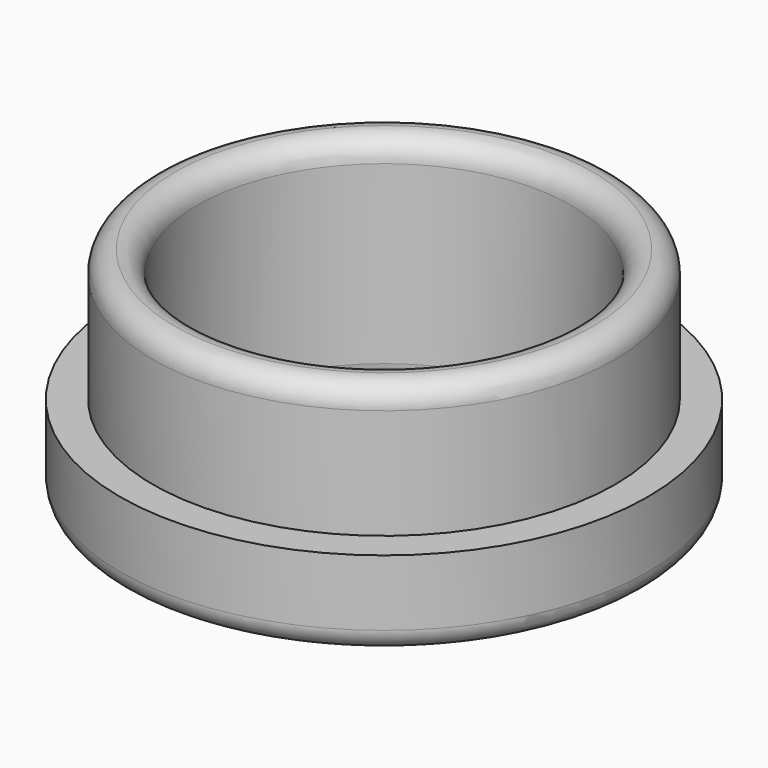
from build123d import *

# Parameters (mm, degrees)
F0_R     = 10.5
F0_R_2   = 8.5
F1_DEPTH = 10
F0_R_3   = 12
F2_DEPTH = 4
F3_R     = 0.99999


# Not quite as in the source:
# - a fillet or chamfer is up to 0.001 mm smaller than in the source, because OpenCascade refuses the exact size


with BuildPart() as f1:
    # F0 (on Top) → F1 (new body)
    with BuildSketch(Plane.XY):
        Circle(F0_R)
        Circle(F0_R_2, mode=Mode.SUBTRACT)
    extrude(amount=F1_DEPTH)

    # F0 (on Top) → F2 (join)
    with BuildSketch(Plane.XY):
        Circle(F0_R_3)
        Circle(F0_R, mode=Mode.SUBTRACT)
    extrude(amount=F2_DEPTH)

    # F3 (radius 1 in the source; OpenCascade refuses exactly that, so slightly less here)
    f3_edges = [f1.edges().sort_by_distance(p)[0] for p in [
        (-8.5, 0, 0),
        (-12, 0, 0),
        (-8.5, 0, 10),
        (-10.5, 0, 10),
    ]]
    fillet(f3_edges, radius=F3_R)


solid = f1.part
